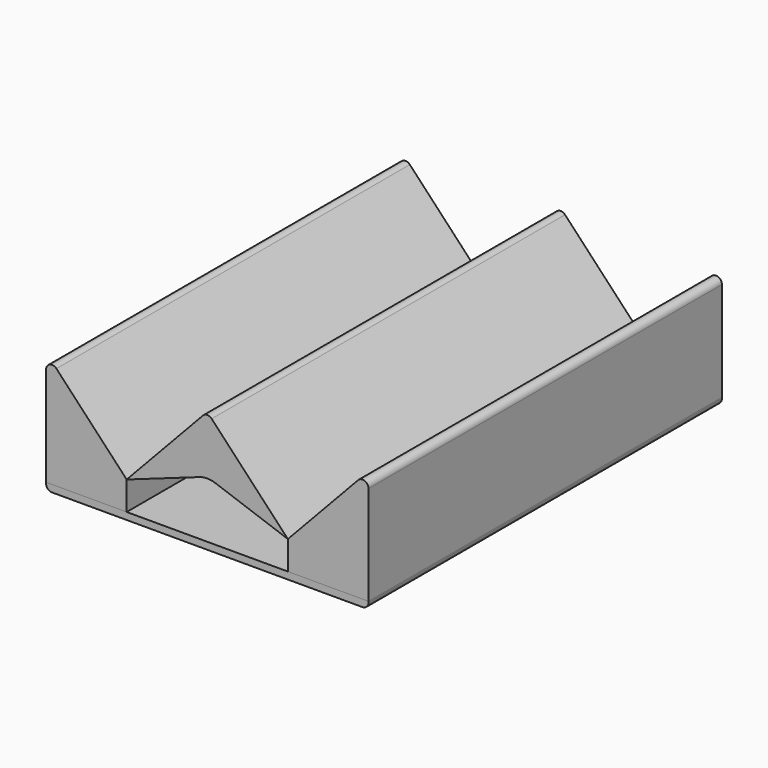
from build123d import *

# Parameters (mm, degrees)
F1_DEPTH = 93.98
F3_DEPTH = 93.98
F4_R     = 5.08
F5_R     = 1.27
F6_R     = 1.27
F6_2_R   = 1.27
F6_3_R   = 1.27


# Not quite as in the source:
# - the program builds the solid bodies; features that only make, move or delete a surface that nothing else refers to are left out


with BuildPart() as f1:
    # F0 (on Front) → F1 (new body)
    with BuildSketch(Plane.XZ):
        Polygon((-17.145, -6.0804947455), (-34.29, 12.160989491), (-34.29, -12.160989491), align=None)
        Polygon((-17.145, -6.0804947455), (-34.29, -12.160989491), (-17.145, -12.160989491), align=None)
    extrude(amount=F1_DEPTH)

    # F5
    f5_edges = [f1.edges().sort_by_distance(p)[0] for p in [
        (-34.29, -46.99, 12.160989),
    ]]
    fillet(f5_edges, radius=F5_R)


with BuildPart() as f1b:
    # F0 (on Front) → F1, piece 2 (new body)
    with BuildSketch(Plane.XZ):
        Polygon((34.29, -12.160989491), (17.145, -6.0804947455), (17.145, -12.160989491), align=None)
        Polygon((34.29, -12.160989491), (34.29, 12.160989491), (17.145, -6.0804947455), align=None)
    extrude(amount=F1_DEPTH)

    # F6
    f6_edges = [f1b.edges().sort_by_distance(p)[0] for p in [
        (34.29, -46.99, 12.160989),
    ]]
    fillet(f6_edges, radius=F6_R)


with BuildPart() as f1c:
    # F0 (on Front) → F1, piece 3 (new body)
    with BuildSketch(Plane.XZ):
        Polygon((17.145, -6.0804947455), (0, 12.160989491), (-17.145, -6.0804947455), (0, 0), align=None)
    extrude(amount=F1_DEPTH)

    # F4
    f4_edges = [f1c.edges().sort_by_distance(p)[0] for p in [
        (0, -46.99, 0),
    ]]
    fillet(f4_edges, radius=F4_R)

    # F6#2
    f6_2_edges = [f1c.edges().sort_by_distance(p)[0] for p in [
        (0, -46.99, 12.160989),
    ]]
    fillet(f6_2_edges, radius=F6_2_R)


with BuildPart() as f3:
    # F0 (on Front) → F3 (new body)
    with BuildSketch(Plane.XZ):
        Polygon((-17.145, -12.160989491), (-34.29, -12.160989491), (-34.29, -13.663481921), (34.29, -13.663481921), (34.29, -12.160989491), (17.145, -12.160989491), align=None)
    extrude(amount=F3_DEPTH)

    # F6#3
    f6_3_edges = [f3.edges().sort_by_distance(p)[0] for p in [
        (-34.29, -46.99, -13.663482),
        (34.29, -46.99, -13.663482),
    ]]
    fillet(f6_3_edges, radius=F6_3_R)


solid = Compound([f1.part, f1b.part, f1c.part, f3.part])
